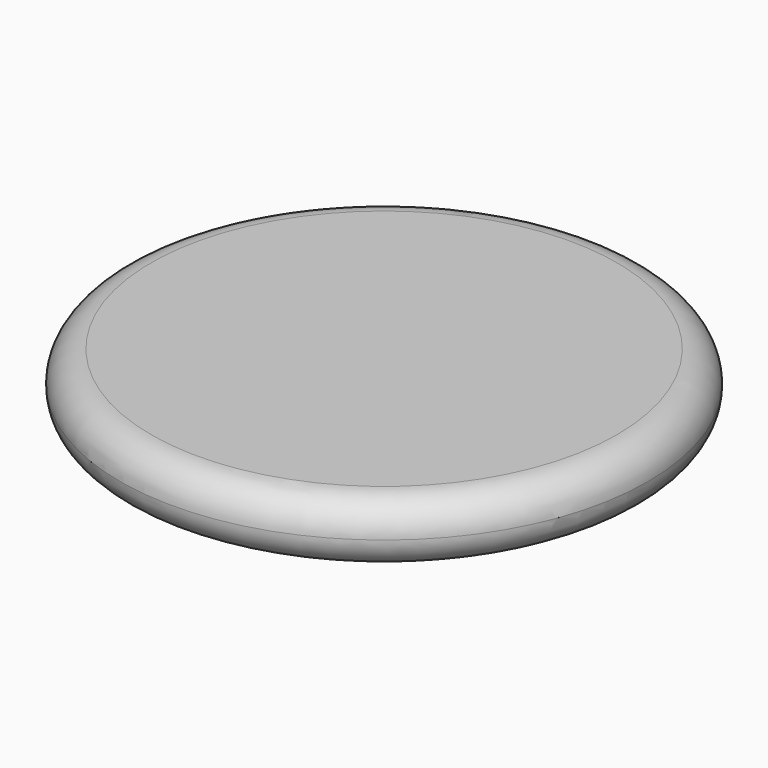
from build123d import *

# Parameters (mm, degrees)
F0_R     = 53.975
F1_DEPTH = 12.7
F2_R     = 6.34999
F3_DEPTH = 10.16
F4_R     = 1.27


# Not quite as in the source:
# - a fillet or chamfer is up to 0.001 mm smaller than in the source, because OpenCascade refuses the exact size


with BuildPart() as f1:
    # F0 (on Top) → F1 (new body)
    with BuildSketch(Plane.XY):
        Circle(F0_R)
    extrude(amount=F1_DEPTH)

    # F2 (radius 6.35 in the source; OpenCascade refuses exactly that, so slightly less here)
    f2_edges = [f1.edges().sort_by_distance(p)[0] for p in [
        (53.975, 0, 6.35),
        (-53.975, 0, 0),
        (-53.975, 0, 12.7),
    ]]
    fillet(f2_edges, radius=F2_R)

    # F3 (cut): a face of the model
    f3_faces = [f1.faces().sort_by_distance(p)[0] for p in [
        (0, 0, 0),
    ]]
    extrude(f3_faces, amount=-F3_DEPTH, mode=Mode.SUBTRACT)

    # F4
    f4_edges = [f1.edges().sort_by_distance(p)[0] for p in [
        (-47.62501, 0, 10.16),
    ]]
    fillet(f4_edges, radius=F4_R)


solid = f1.part
